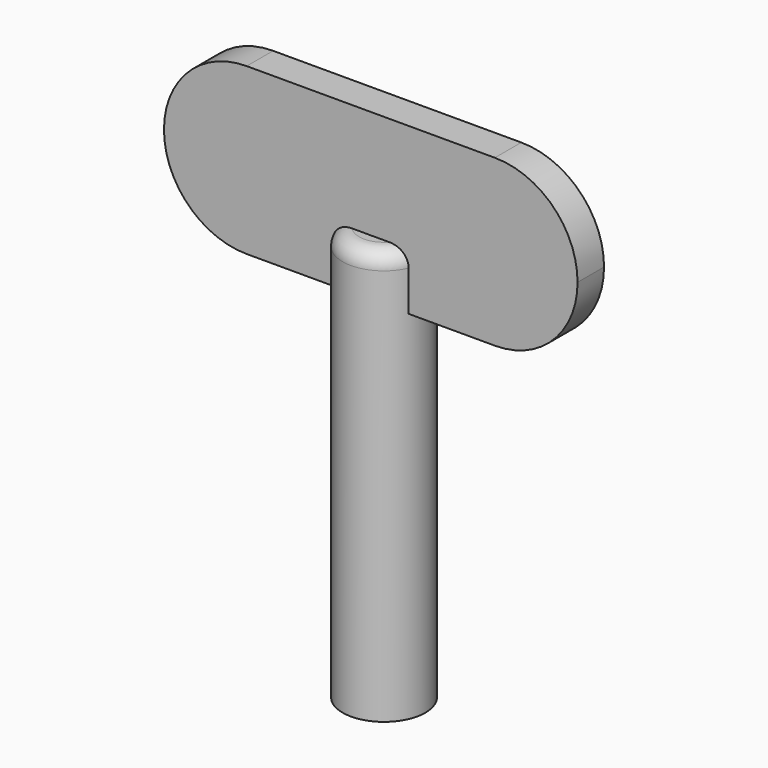
from build123d import *

# Parameters (mm, degrees)
F0_R     = 2.5
F0_R_2   = 1.01
F1_DEPTH = 25
F2_W     = 25
F2_H     = 10
F3_DEPTH = 1
F4_R     = 4.99999
F5_R     = 1


# Not quite as in the source:
# - a fillet or chamfer is up to 0.001 mm smaller than in the source, because OpenCascade refuses the exact size


with BuildPart() as f1:
    # F0 (on Top) → F1 (new body)
    with BuildSketch(Plane.XY):
        Circle(F0_R)
        Circle(F0_R_2, mode=Mode.SUBTRACT)
    extrude(amount=F1_DEPTH)

    # F2 (on Front) → F3 (join, symmetric)
    with BuildSketch(Plane.XZ):
        with Locations((0, 26.5656393021)):
            Rectangle(F2_W, F2_H)
    extrude(amount=F3_DEPTH, both=True)

    # F4 (radius 5 in the source; OpenCascade refuses exactly that, so slightly less here)
    f4_edges = [f1.edges().sort_by_distance(p)[0] for p in [
        (-12.5, 0, 21.565639),
        (-12.5, 0, 31.565639),
        (12.5, 0, 21.565639),
        (12.5, 0, 31.565639),
    ]]
    fillet(f4_edges, radius=F4_R)

    # F5
    f5_edges = [f1.edges().sort_by_distance(p)[0] for p in [
        (0, 2.5, 25),
        (0, -2.5, 25),
    ]]
    fillet(f5_edges, radius=F5_R)


solid = f1.part
